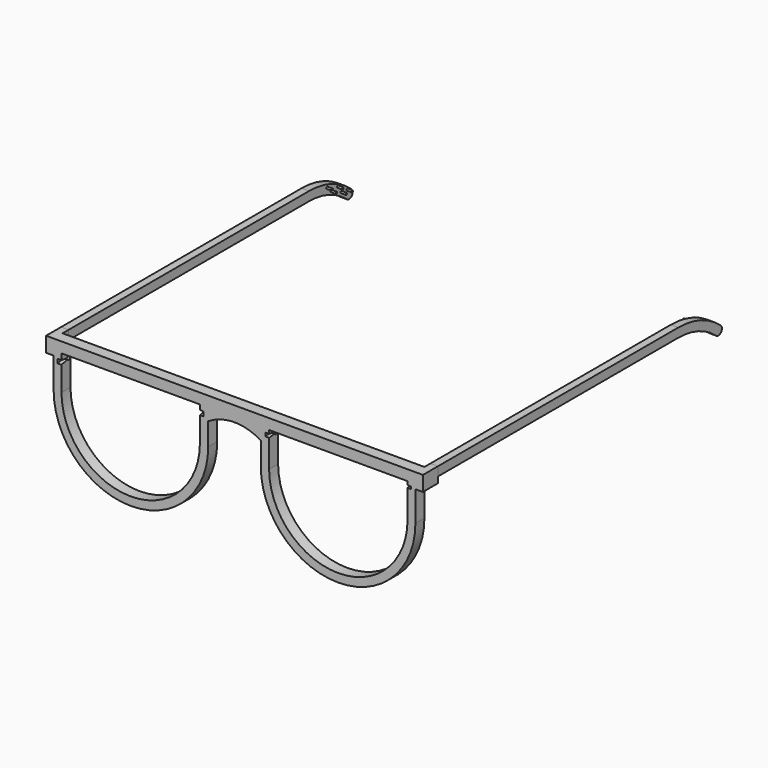
from build123d import *

# Parameters (mm, degrees)
F1_DEPTH  = 3.81
F2_W      = 6.35
F2_H      = 5.08
F3_DEPTH  = 2.54
F5_W      = 101.6
F5_H      = 3.048
F6_DEPTH  = 2.54
F7_W      = 101.6
F7_H      = 2.54
F8_DEPTH  = 2.54
F9_W      = 20.4162850118
F9_H      = 1.9500367343
F10_DEPTH = 0.254
F12_DEPTH = 2.54
F14_R     = 0.3175
F15_DEPTH = 1.778
F18_DEPTH = 1.143
F20_DEPTH = 1.27
F22_DEPTH = 1.27
F24_DEPTH = 1.27


with BuildPart() as f1:
    # F0 (on Front) → F1 (new body)
    with BuildSketch(Plane.XZ):
        with BuildLine():
            Line((8.89, 35.491819303), (0, 35.491819303))
            Line((0, 35.491819303), (-8.89, 35.491819303))
            Line((-8.89, 35.491819303), (-8.89, 27.8771001825))
            ThreePointArc((-8.89, 27.8771001825), (0, 30.4448411771), (8.89, 27.8771001825))
            Line((8.89, 27.8771001825), (8.89, 35.491819303))
        make_face()
        with BuildLine():
            Line((-8.89, 27.8771001825), (-8.89, 35.491819303))
            Line((-8.89, 35.491819303), (-61.167026878, 35.491819303))
            Line((-61.167026878, 35.491819303), (-61.167026878, 20.2623810619))
            ThreePointArc((-61.167026878, 20.2623810619), (-35.028513439, -5.8761323771), (-8.89, 20.2623810619))
            Line((-8.89, 20.2623810619), (-8.89, 27.8771001825))
        make_face()
        with BuildLine():
            ThreePointArc((-11.7025515065, 20.2623810619), (-35.1013853215, -3.0397615448), (-58.5002191365, 20.2623810619))
            Line((-58.5002191365, 20.2623810619), (-58.5002191365, 31.9472067058))
            Line((-58.5002191365, 31.9472067058), (-11.7025515065, 31.9472067058))
            Line((-11.7025515065, 31.9472067058), (-11.7025515065, 20.2623810619))
        make_face(mode=Mode.SUBTRACT)
        with BuildLine():
            Line((61.167026878, 35.491819303), (8.89, 35.491819303))
            Line((8.89, 35.491819303), (8.89, 27.8771001825))
            Line((8.89, 27.8771001825), (8.89, 20.2623810619))
            ThreePointArc((8.89, 20.2623810619), (35.028513439, -5.8761323771), (61.167026878, 20.2623810619))
            Line((61.167026878, 20.2623810619), (61.167026878, 35.491819303))
        make_face()
        with BuildLine():
            Line((11.7025515065, 31.9472067058), (58.5002191365, 31.9472067058))
            Line((58.5002191365, 31.9472067058), (58.5002191365, 20.2623810619))
            ThreePointArc((58.5002191365, 20.2623810619), (35.1013853215, -3.0397615448), (11.7025515065, 20.2623810619))
            Line((11.7025515065, 20.2623810619), (11.7025515065, 31.9472067058))
        make_face(mode=Mode.SUBTRACT)
    extrude(amount=F1_DEPTH)

    # F2 (on face) → F3 (join)
    with BuildSketch(Plane.YZ.offset(61.167026878)):
        with Locations((-0.635, 32.951819303)):
            Rectangle(F2_W, F2_H)
    extrude(amount=F3_DEPTH)

    # F4: F1 across plane


with BuildPart() as f1_1:
    add(f1.part)
    add(f1.part.mirror(Plane.YZ))

    # F17 (on face) → F18 (cut)
    with BuildSketch(Plane(origin=(58.5002191365, 0, 0), x_dir=(0, -1, 0), z_dir=(-1, 0, 0))):
        with BuildLine():
            ThreePointArc((1.2845198591, 30.239206098), (1.2988156365, 30.2992732373), (1.303619671, 30.3608309478))
            ThreePointArc((1.303619671, 30.3608309478), (1.2874340011, 30.4730040235), (1.2401974525, 30.5760257848))
            ThreePointArc((1.2401974525, 30.5760257848), (0.5134218421, 30.3090626702), (1.2845198591, 30.239206098))
        make_face()
        with BuildLine():
            ThreePointArc((1.2401974525, 30.5760257848), (1.2874340011, 30.4730040235), (1.303619671, 30.3608309478))
            ThreePointArc((1.303619671, 30.3608309478), (1.2988156365, 30.2992732373), (1.2845198591, 30.239206098))
            Line((1.2845198591, 30.239206098), (3.81, 29.9640362842))
            Line((3.81, 29.9640362842), (3.81, 30.7576256113))
            Line((3.81, 30.7576256113), (1.2401974525, 30.5760257848))
        make_face()
    extrude(amount=-F18_DEPTH, mode=Mode.SUBTRACT)

    # F19 (on face) → F20 (cut)
    with BuildSketch(Plane.YZ.offset(11.7025515065)):
        with BuildLine():
            ThreePointArc((-1.5344448459, 29.9096479588), (-0.843178998, 29.5043172702), (-0.3267133253, 30.1170200109))
            ThreePointArc((-0.3267133253, 30.1170200109), (-0.771947349, 30.7131266136), (-1.469903859, 30.455380367))
            ThreePointArc((-1.469903859, 30.455380367), (-1.5657489749, 30.1900328091), (-1.5344448459, 29.9096479588))
        make_face()
        with BuildLine():
            ThreePointArc((-1.5344448459, 29.9096479588), (-1.5657489749, 30.1900328091), (-1.469903859, 30.455380367))
            Line((-1.469903859, 30.455380367), (-3.81, 30.7979229838))
            Line((-3.81, 30.7979229838), (-3.81, 29.607038945))
            Line((-3.81, 29.607038945), (-1.5344448459, 29.9096479588))
        make_face()
    extrude(amount=-F20_DEPTH, mode=Mode.SUBTRACT)

    # F21 (on face) → F22 (cut)
    with BuildSketch(Plane.YZ.offset(-58.5002191365)):
        with BuildLine():
            ThreePointArc((-1.3648844893, 29.0673966875), (-0.6670225121, 28.7422296785), (-0.189563217, 29.3461978436))
            ThreePointArc((-0.189563217, 29.3461978436), (-0.707470296, 29.9583508822), (-1.3969558464, 29.5489992474))
            ThreePointArc((-1.3969558464, 29.5489992474), (-1.4296478817, 29.304953043), (-1.3648844893, 29.0673966875))
        make_face()
        with BuildLine():
            ThreePointArc((-1.3648844893, 29.0673966875), (-1.4296478817, 29.304953043), (-1.3969558464, 29.5489992474))
            Line((-1.3969558464, 29.5489992474), (-3.81, 29.9056489021))
            Line((-3.81, 29.9056489021), (-3.81, 28.5336878151))
            Line((-3.81, 28.5336878151), (-1.3648844893, 29.0673966875))
        make_face()
    extrude(amount=-F22_DEPTH, mode=Mode.SUBTRACT)

    # F23 (on face) → F24 (cut)
    with BuildSketch(Plane(origin=(-11.7025515065, 0, 0), x_dir=(0, -1, 0), z_dir=(-1, 0, 0))):
        with BuildLine():
            ThreePointArc((1.3434285805, 29.2105876086), (1.4150944565, 29.3721062282), (1.4396124445, 29.5471008867))
            ThreePointArc((1.4396124445, 29.5471008867), (1.4265256847, 29.6755339351), (1.3878033244, 29.7986878633))
            ThreePointArc((1.3878033244, 29.7986878633), (0.1678927477, 29.5950112055), (1.3434285805, 29.2105876086))
        make_face()
        with BuildLine():
            ThreePointArc((1.3878033244, 29.7986878633), (1.4265256847, 29.6755339351), (1.4396124445, 29.5471008867))
            ThreePointArc((1.4396124445, 29.5471008867), (1.4150944565, 29.3721062282), (1.3434285805, 29.2105876086))
            Line((1.3434285805, 29.2105876086), (3.81, 28.7525691092))
            Line((3.81, 28.7525691092), (3.81, 30.2800890058))
            Line((3.81, 30.2800890058), (1.3878033244, 29.7986878633))
        make_face()
    extrude(amount=-F24_DEPTH, mode=Mode.SUBTRACT)


with BuildPart() as f6:
    # F5 (on face) → F6 (new body)
    with BuildSketch(Plane.YZ.offset(63.707026878)):
        with Locations((53.34, 33.967819303)):
            Rectangle(F5_W, F5_H)
    extrude(amount=-F6_DEPTH)

    # F11 (on face) → F12 (join)
    with BuildSketch(Plane.YZ.offset(63.707026878)):
        with BuildLine():
            ThreePointArc((104.14, 32.443819303), (112.6305060514, 30.9330988595), (120.0787946582, 26.5863798559))
            ThreePointArc((120.0787946582, 26.5863798559), (122.210042136, 26.7338822785), (122.0027580857, 28.8601480424))
            ThreePointArc((122.0027580857, 28.8601480424), (113.667029838, 33.780400665), (104.14, 35.491819303))
            Line((104.14, 35.491819303), (104.14, 32.443819303))
        make_face()
    extrude(amount=-F12_DEPTH)


with BuildPart() as f8:
    # F7 (on face) → F8 (new body)
    with BuildSketch(Plane(origin=(-63.707026878, 0, 0), x_dir=(0, -1, 0), z_dir=(-1, 0, 0))):
        with Locations((-53.34, 34.221819303)):
            Rectangle(F7_W, F7_H)
    extrude(amount=-F8_DEPTH)


with BuildPart() as f10:
    # F9 (on face) → F10 (new body)
    with BuildSketch(Plane(origin=(-63.707026878, 0, 0), x_dir=(0, -1, 0), z_dir=(-1, 0, 0))):
        with Locations((-63.5481425059, 34.3102347106)):
            Rectangle(F9_W, F9_H)
    extrude(amount=F10_DEPTH)


with BuildPart() as f13_1:
    # F13: instance of F6
    add(f6.part.mirror(Plane.YZ))

    # F16: F15d, F15e, F15b, F15, F15c across plane


with BuildPart() as f15:
    # F14 (on face) → F15 (new body)
    with BuildSketch(Plane(origin=(61.167026878, 0, 0), x_dir=(0, -1, 0), z_dir=(-1, 0, 0))):
        with Locations((-120.2708929777, 29.4003784657)):
            Circle(F14_R)
    extrude(amount=F15_DEPTH)


with BuildPart() as f15b:
    # F14 (on face) → F15, piece 2 (new body)
    with BuildSketch(Plane(origin=(61.167026878, 0, 0), x_dir=(0, -1, 0), z_dir=(-1, 0, 0))):
        with Locations((-117.7130416036, 29.7041404992)):
            Circle(F14_R)
    extrude(amount=F15_DEPTH)


with BuildPart() as f15c:
    # F14 (on face) → F15, piece 3 (new body)
    with BuildSketch(Plane(origin=(61.167026878, 0, 0), x_dir=(0, -1, 0), z_dir=(-1, 0, 0))):
        with Locations((-116.2837222219, 31.8854898214)):
            Circle(F14_R)
    extrude(amount=F15_DEPTH)


with BuildPart() as f15d:
    # F14 (on face) → F15, piece 4 (new body)
    with BuildSketch(Plane(origin=(61.167026878, 0, 0), x_dir=(0, -1, 0), z_dir=(-1, 0, 0))):
        with Locations((-113.4407967329, 31.7698046565)):
            Circle(F14_R)
    extrude(amount=F15_DEPTH)


with BuildPart() as f15e:
    # F14 (on face) → F15, piece 5 (new body)
    with BuildSketch(Plane(origin=(61.167026878, 0, 0), x_dir=(0, -1, 0), z_dir=(-1, 0, 0))):
        with Locations((-111.7342412472, 33.3984978497)):
            Circle(F14_R)
    extrude(amount=F15_DEPTH)


with BuildPart() as f13_1_1:
    add(f13_1.part)
    add(f15d.part.mirror(Plane.YZ))
    add(f15e.part.mirror(Plane.YZ))
    add(f15b.part.mirror(Plane.YZ))
    add(f15.part.mirror(Plane.YZ))
    add(f15c.part.mirror(Plane.YZ))


solid = Compound([f1_1.part, f6.part, f8.part, f10.part, f15.part, f15b.part, f15c.part, f15d.part, f15e.part, f13_1_1.part])
